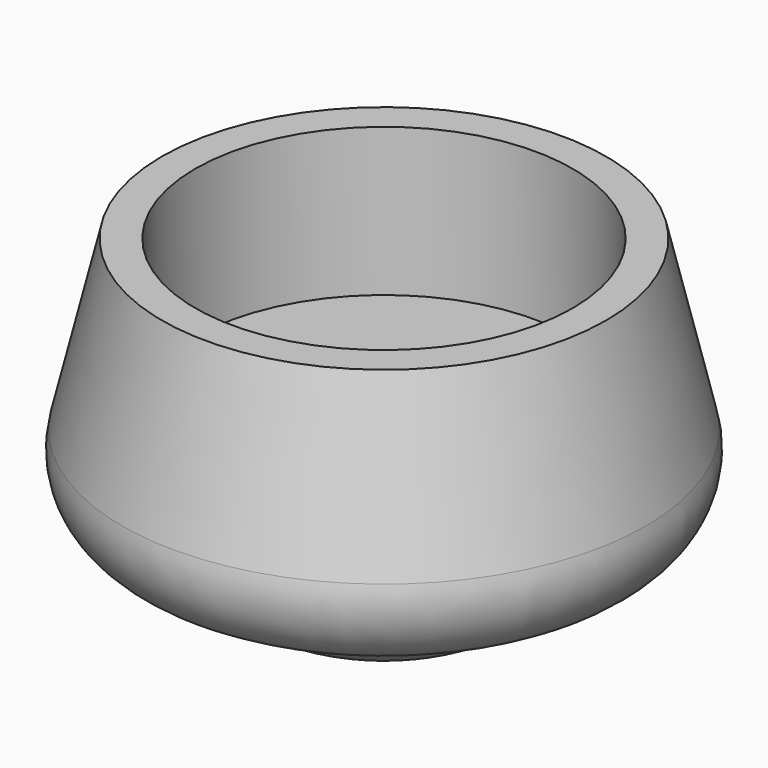
from build123d import *

# Parameters (mm, degrees)
F0_R     = 7.6617406775
F2_R     = 6
F4_R     = 2
F5_R     = 4.7899887375
F6_DEPTH = 2
F8_R     = 5.1
F9_DEPTH = 4


# Not quite as in the source:
# - a fillet or chamfer that OpenCascade refuses, or shapes differently, is made with other operations: its cross-section is extruded or revolved along the edge and cut away or added


with BuildPart() as f3:
    # F0 (on Top) → F3 section 0
    with BuildSketch(Plane.XY):
        Circle(F0_R)
    # F2 (on offset) → F3 section 1
    with BuildSketch(Plane.XY.offset(7)):
        Circle(F2_R)
    loft()

    # F4
    f4_edges = [f3.edges().sort_by_distance(p)[0] for p in [
        (-7.661741, 0, 0),
    ]]
    fillet(f4_edges, radius=F4_R)

    # F5 (on face) → F6 (join)
    with BuildSketch(Plane(origin=(0, 0, 0), x_dir=(1, 0, 0), z_dir=(0, 0, -1))):
        Circle(F5_R)
    extrude(amount=F6_DEPTH)

    # F7: fillet of radius 5 on 1 edges, made by hand

    # F7_s1 → F7_t2 (revolve, cut)
    with BuildSketch(Plane.XZ):
        with BuildLine():
            ThreePointArc((4.7899887375, 0), (3.026056715, -1.472135955), (0.7899887375, -2))
            Line((0.7899887375, -2), (4.7899887375, -2))
            Line((4.7899887375, -2), (4.7899887375, 0))
        make_face()
    revolve(axis=Axis((0, 0, -2), (0, 0, -1)), mode=Mode.SUBTRACT)

    # F8 (on face) → F9 (cut)
    with BuildSketch(Plane.XY.offset(7)):
        Circle(F8_R)
    extrude(amount=-F9_DEPTH, mode=Mode.SUBTRACT)


solid = f3.part
